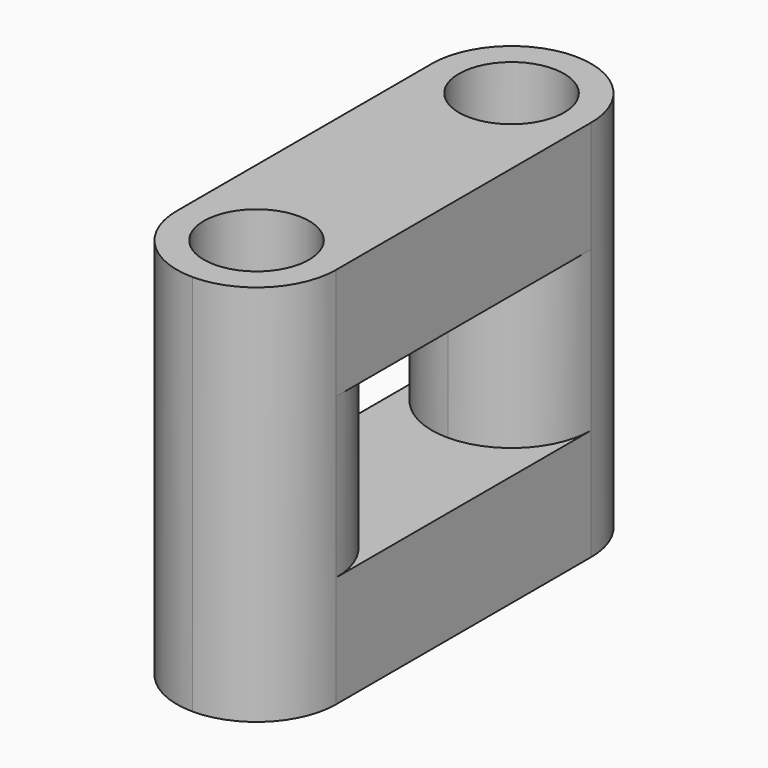
from build123d import *

# Parameters (mm, degrees)
F0_W     = 5
F0_H     = 15
F1_DEPTH = 12
F2_W     = 5
F2_H     = 5
F3_DEPTH = 5
F4_R     = 2.49999
F6_D     = 3.3


# Not quite as in the source:
# - a fillet or chamfer is up to 0.001 mm smaller than in the source, because OpenCascade refuses the exact size


with BuildPart() as f1:
    # F0 (on Top) → F1 (new body)
    with BuildSketch(Plane.XY):
        Rectangle(F0_W, F0_H)
    extrude(amount=F1_DEPTH)

    # F2 (on face) → F3 (cut, through all)
    with BuildSketch(Plane.YZ.offset(2.5)):
        with Locations((0, 6)):
            Rectangle(F2_W, F2_H)
    extrude(amount=-F3_DEPTH, mode=Mode.SUBTRACT)

    # F4 (radius 2.5 in the source; OpenCascade refuses exactly that, so slightly less here)
    f4_edges = [f1.edges().sort_by_distance(p)[0] for p in [
        (2.5, -7.5, 6),
        (-2.5, -7.5, 6),
        (2.5, 7.5, 6),
        (-2.5, 7.5, 6),
        (-2.5, 2.5, 6),
        (-2.5, -2.5, 6),
        (2.5, -2.5, 6),
        (2.5, 2.5, 6),
    ]]
    fillet(f4_edges, radius=F4_R)

    # F6 (through all)
    with Locations(Plane.XY.offset(12)):
        with Locations((0, 5), (0, -5)):
            Hole(F6_D / 2)


solid = f1.part
